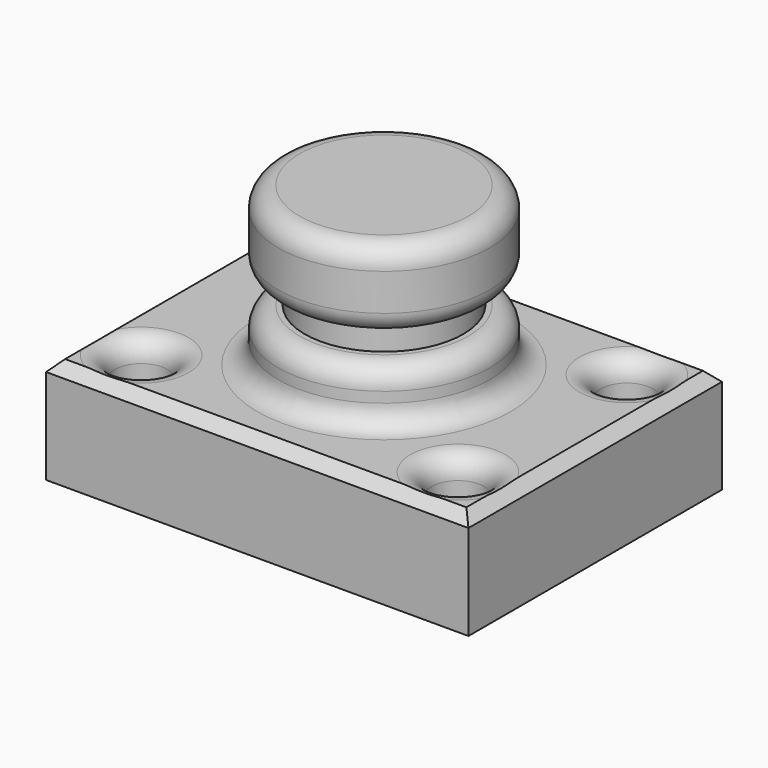
from build123d import *

# Parameters (mm, degrees)
F0_W          = 101.6
F0_H          = 76.2
F1_DEPTH      = 25.4
F2_R          = 6.35
F3_DEPTH      = 25.4
F3_DEPTH_BACK = 25.4
F4_W          = 25.4
F4_H          = 38.1
F6_W          = 19.05
F6_H          = 6.35
F8_SIZE       = 2.54
F9_R          = 5.08


# Not quite as in the source:
# - a fillet or chamfer that OpenCascade refuses, or shapes differently, is made with other operations: its cross-section is extruded or revolved along the edge and cut away or added


with BuildPart() as f1:
    # F0 (on Top) → F1 (new body)
    with BuildSketch(Plane.XY):
        Rectangle(F0_W, F0_H)
    extrude(amount=F1_DEPTH)

    # F2 (on Top) → F3 (cut, two sides)
    with BuildSketch(Plane.XY) as f3_sk:
        with Locations((-38.1, 25.4)):
            Circle(F2_R)
        with Locations((38.1, 25.4)):
            Circle(F2_R)
        with Locations((-38.1, -25.4)):
            Circle(F2_R)
        with Locations((38.1, -25.4)):
            Circle(F2_R)
    extrude(amount=-F3_DEPTH, mode=Mode.SUBTRACT)
    extrude(f3_sk.sketch, amount=F3_DEPTH_BACK, mode=Mode.SUBTRACT)

    # F4 (on Front) → F5 (revolve)
    with BuildSketch(Plane.XZ):
        with Locations((12.7, 44.45)):
            Rectangle(F4_W, F4_H)
    revolve(axis=Axis((0, 0, 44.45), (0, 0, -1)))

    # F6 (on Right) → F7 (revolve, cut)
    with BuildSketch(Plane.YZ):
        with Locations((-28.575, 41.275)):
            Rectangle(F6_W, F6_H)
    revolve(axis=Axis((0, 0, 25.4), (0, 0, 1)), mode=Mode.SUBTRACT)

    # F8
    f8_edges = [f1.edges().sort_by_distance(p)[0] for p in [
        (0, -38.1, 25.4),
        (-50.8, 0, 25.4),
        (0, 38.1, 25.4),
        (50.8, 0, 25.4),
    ]]
    chamfer(f8_edges, length=F8_SIZE)

    # F9
    f9_edges = [f1.edges().sort_by_distance(p)[0] for p in [
        (-25.4, 0, 25.4),
        (-25.4, 0, 44.45),
        (-25.4, 0, 38.1),
        (-25.4, 0, 63.5),
    ]]
    fillet(f9_edges, radius=F9_R)

    # F10: fillet of radius 5.08 on 9 edges, made by hand

    # F10_s1 → F10_t2 (revolve, cut)
    with BuildSketch(Plane.XZ.offset(-25.4)):
        with BuildLine():
            ThreePointArc((49.53, 25.4), (45.9378975516, 23.9121024484), (44.45, 20.32))
            Line((44.45, 20.32), (44.45, 25.4))
            Line((44.45, 25.4), (49.53, 25.4))
        make_face()
    revolve(axis=Axis((38.1, 25.4, 25.4), (0, 0, 1)), mode=Mode.SUBTRACT)

    # F10_s3 → F10_t4 (revolve, cut)
    with BuildSketch(Plane.XZ.offset(25.4)):
        with BuildLine():
            ThreePointArc((49.53, 25.4), (45.9378975516, 23.9121024484), (44.45, 20.32))
            Line((44.45, 20.32), (44.45, 25.4))
            Line((44.45, 25.4), (49.53, 25.4))
        make_face()
    revolve(axis=Axis((38.1, -25.4, 25.4), (0, 0, 1)), mode=Mode.SUBTRACT)

    # F10_s5 → F10_t6 (revolve, cut)
    with BuildSketch(Plane.XZ.offset(25.4)):
        with BuildLine():
            ThreePointArc((-26.67, 25.4), (-30.2621024484, 23.9121024484), (-31.75, 20.32))
            Line((-31.75, 20.32), (-31.75, 25.4))
            Line((-31.75, 25.4), (-26.67, 25.4))
        make_face()
    revolve(axis=Axis((-38.1, -25.4, 25.4), (0, 0, 1)), mode=Mode.SUBTRACT)

    # F10_s7 → F10_t8 (revolve, cut)
    with BuildSketch(Plane.XZ.offset(-25.4)):
        with BuildLine():
            ThreePointArc((-26.67, 25.4), (-30.2621024484, 23.9121024484), (-31.75, 20.32))
            Line((-31.75, 20.32), (-31.75, 25.4))
            Line((-31.75, 25.4), (-26.67, 25.4))
        make_face()
    revolve(axis=Axis((-38.1, 25.4, 25.4), (0, 0, 1)), mode=Mode.SUBTRACT)

    # F10_s9 → F10_t10 (revolve, cut)
    with BuildSketch(Plane.XZ.offset(-25.4)):
        with BuildLine():
            ThreePointArc((44.45, 5.08), (45.9378975516, 1.4878975516), (49.53, 0))
            Line((49.53, 0), (44.45, 0))
            Line((44.45, 0), (44.45, 5.08))
        make_face()
    revolve(axis=Axis((38.1, 25.4, 0), (0, 0, 1)), mode=Mode.SUBTRACT)

    # F10_s11 → F10_t12 (revolve, cut)
    with BuildSketch(Plane.XZ.offset(25.4)):
        with BuildLine():
            ThreePointArc((44.45, 5.08), (45.9378975516, 1.4878975516), (49.53, 0))
            Line((49.53, 0), (44.45, 0))
            Line((44.45, 0), (44.45, 5.08))
        make_face()
    revolve(axis=Axis((38.1, -25.4, 0), (0, 0, 1)), mode=Mode.SUBTRACT)

    # F10_s13 → F10_t14 (revolve, cut)
    with BuildSketch(Plane.XZ.offset(25.4)):
        with BuildLine():
            ThreePointArc((-31.75, 5.08), (-30.2621024484, 1.4878975516), (-26.67, 0))
            Line((-26.67, 0), (-31.75, 0))
            Line((-31.75, 0), (-31.75, 5.08))
        make_face()
    revolve(axis=Axis((-38.1, -25.4, 0), (0, 0, 1)), mode=Mode.SUBTRACT)

    # F10_s15 → F10_t16 (revolve, cut)
    with BuildSketch(Plane.XZ.offset(-25.4)):
        with BuildLine():
            ThreePointArc((-31.75, 5.08), (-30.2621024484, 1.4878975516), (-26.67, 0))
            Line((-26.67, 0), (-31.75, 0))
            Line((-31.75, 0), (-31.75, 5.08))
        make_face()
    revolve(axis=Axis((-38.1, 25.4, 0), (0, 0, 1)), mode=Mode.SUBTRACT)


solid = f1.part
